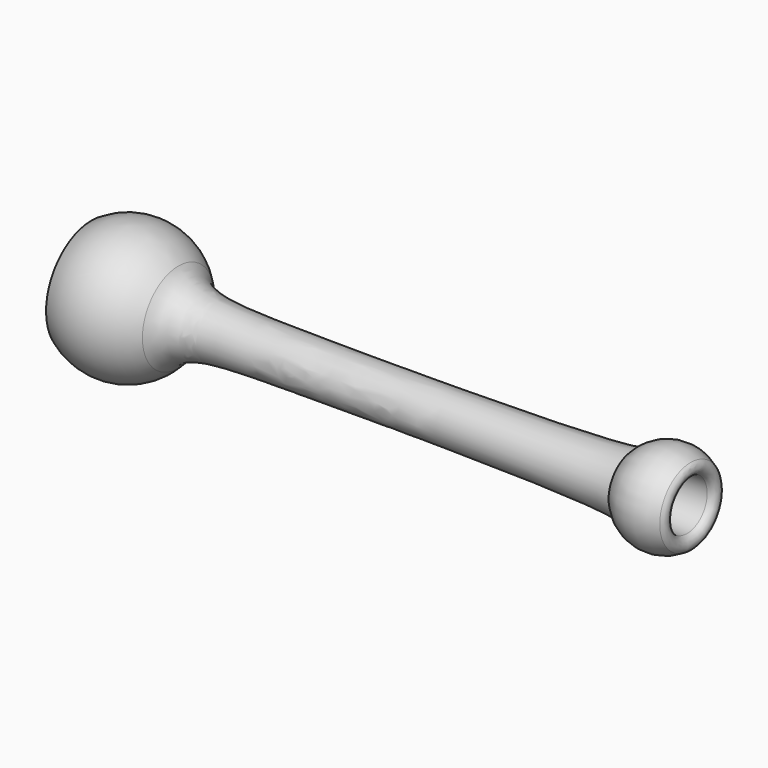
from build123d import *

# Parameters (mm, degrees)
F2_R = 2


# Not quite as in the source:
# - a fillet or chamfer that OpenCascade refuses, or shapes differently, is made with other operations: its cross-section is extruded or revolved along the edge and cut away or added


with BuildPart() as f1:
    # F0 (on Front) → F1 (revolve)
    with BuildSketch(Plane.XZ):
        with BuildLine():
            ThreePointArc((-7.0685046336, 10.3095219212), (4.6853520259, 11.5886788028), (12.2474487139, 2.5))
            Line((12.2474487139, 2.5), (74.2474487139, 2.5))
            Line((74.2474487139, 2.5), (157.3572822072, 7.1481325134))
            ThreePointArc((157.3572822072, 7.1481325134), (148.0868112725, 12.5485391429), (138.2025005846, 8.3764383123))
            add(Edge.make_bspline(
                [(13.7809895682, 12.3177978136), (17.0667820514, 6.8991035875), (43.2053805171, 6.3860439818), (129.6258643455, 6.3638695803), (138.2025005846, 8.3764383123)],
                knots=[0, 0, 0, 0, 0.3640216959, 1, 1, 1, 1], degree=3))
            ThreePointArc((13.7809895682, 12.3177978136), (2.4835532955, 18.3159979112), (-10.003236638, 15.5428141988))
            Line((-10.003236638, 15.5428141988), (-7.0685046336, 10.3095219212))
        make_face()
    revolve(axis=Axis((35, 0, 0), (1, 0, 0)))

    # F2
    f2_edges = [f1.edges().sort_by_distance(p)[0] for p in [
        (157.357282, 0, -7.148133),
        (-7.068505, 0, -10.309522),
        (12.247449, 0, -2.5),
    ]]
    fillet(f2_edges, radius=F2_R)

    # F3: fillet of radius 5 on 1 edges, made by hand

    # F3_s1 → F3_t2 (revolve, cut)
    with BuildSketch(Plane.XZ):
        with BuildLine():
            ThreePointArc((74.3869405319, 2.5078014409), (74.2473942064, 2.5019507408), (74.1077389084, 2.5))
            Line((74.1077389084, 2.5), (74.1077389084, 2.4))
            Line((74.1077389084, 2.4), (74.25024291, 2.4))
            Line((74.25024291, 2.4), (74.3925245643, 2.4079574697))
            Line((74.3925245643, 2.4079574697), (74.3869405319, 2.5078014409))
        make_face()
    revolve(axis=Axis((74.2474487139, 0, 0), (1, 0, 0)), mode=Mode.SUBTRACT)


solid = f1.part
